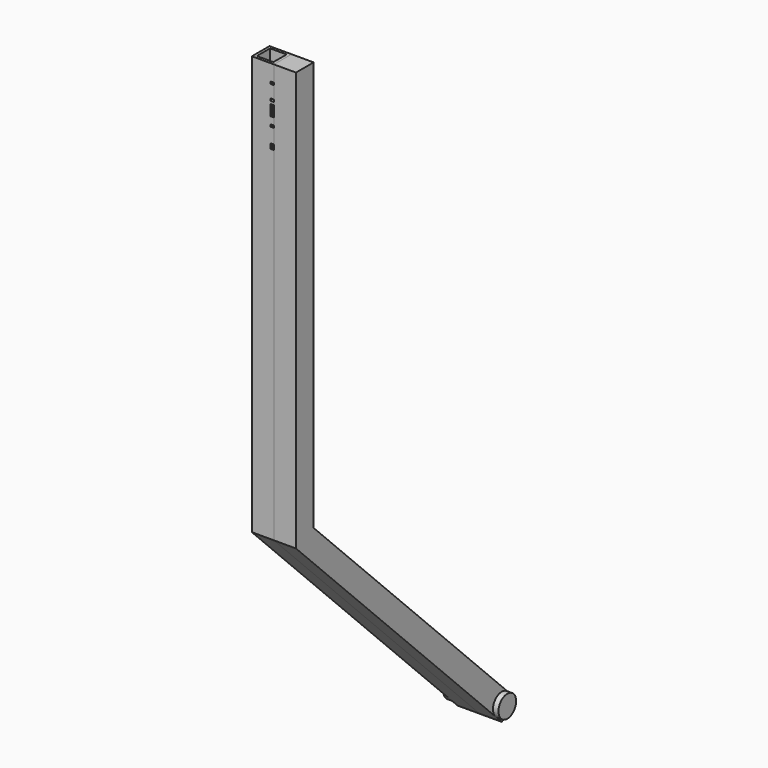
from build123d import *

# Parameters (mm, degrees)
F1_DEPTH     = 20
F3_DEPTH     = 5
F5_W         = 15
F5_H         = 15
F6_DEPTH     = 100
F7_TEXT_SIZE = 24.6410723776
F8_DEPTH     = 3


# Not quite as in the source:
# - Text() gives the source's letters only with a copy of the font that has no kerning and outlines rounded to 1/6400 em; it was checked with that copy


with BuildPart() as f1:
    # F0 (on Right) → F1 (new body)
    with BuildSketch(Plane.YZ):
        Polygon((-53.8653362151, 203.3568546289), (-73.8653362151, 203.3568546289), (-73.8653362151, -176.6431453711), (-53.8653362151, -168.3588741236), align=None)
        Polygon((-53.8653362151, -168.3588741236), (-73.8653362151, -176.6431453711), (159.4799015765, -409.9883831626), (173.6220372002, -395.8462475389), align=None)
    extrude(amount=F1_DEPTH)

    # F2 (on face) → F3 (join)
    with BuildSketch(Plane.YZ.offset(20)):
        with BuildLine():
            ThreePointArc((166.55096926, -402.9173154791), (168.7186968668, -399.6730819464), (169.4799015765, -395.8462475389))
            ThreePointArc((169.4799015765, -395.8462475389), (168.7186969016, -392.0194132152), (166.5509693883, -388.775179727))
            ThreePointArc((166.5509693883, -388.775179727), (152.408833765, -388.7751797267), (152.4088337639, -402.91731535))
            ThreePointArc((152.4088337639, -402.91731535), (159.4799014852, -405.8462475389), (166.55096926, -402.9173154791))
        make_face()
    extrude(amount=F3_DEPTH)


with BuildPart() as f4_1:
    # F4: instance of F1
    add(f1.part.mirror(Plane.YZ))

    # F5 (on face) → F6 (cut)
    with BuildSketch(Plane.XY.offset(203.3568546289)):
        with Locations((-10, -63.8653362151)):
            Rectangle(F5_W, F5_H)
    extrude(amount=-F6_DEPTH, mode=Mode.SUBTRACT)

    # F7 (on face) → F8 (cut)
    with BuildSketch(Plane.YZ):
        with Locations(Location((-73.8653362151, 188.7981017571), (0, 0, -90))):
            Text('ALTO', F7_TEXT_SIZE, font='Open Sans', text_align=(TextAlign.LEFT, TextAlign.BOTTOM))
    extrude(amount=-F8_DEPTH, mode=Mode.SUBTRACT)


solid = Compound([f1.part, f4_1.part])
